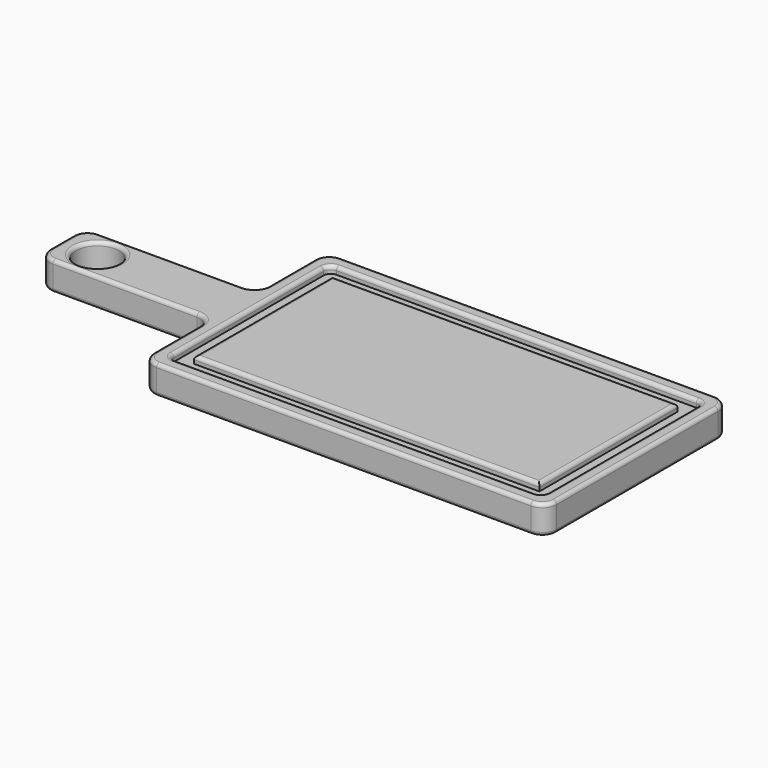
from build123d import *

# Parameters (mm, degrees)
F0_W     = 152.4
F0_H     = 50.8
F1_DEPTH = 25.4
F2_R     = 19.05
F3_DEPTH = 25.4
F5_DEPTH = 6.35
F6_R     = 6.35
F7_R     = 12.7
F8_R     = 12.7
F9_R     = 3.17499


# Not quite as in the source:
# - a fillet or chamfer is up to 0.001 mm smaller than in the source, because OpenCascade refuses the exact size


with BuildPart() as f1:
    # F0 (on Top) → F1 (new body)
    with BuildSketch(Plane.XY):
        Polygon((0, 76.2), (0, 0), (355.6, 0), (355.6, 203.2), (0, 203.2), (0, 127), align=None)
        with Locations((-76.2, 101.6)):
            Rectangle(F0_W, F0_H)
    extrude(amount=F1_DEPTH)

    # F2 (on face) → F3 (cut)
    with BuildSketch(Plane.XY.offset(25.4)):
        with Locations((-120.65, 101.6)):
            Circle(F2_R)
    extrude(amount=-F3_DEPTH, mode=Mode.SUBTRACT)

    # F4 (on face) → F5 (cut)
    with BuildSketch(Plane.XY.offset(25.4)):
        Polygon((12.6999939203, 76.2), (12.6999939203, 12.6999939203), (342.9000060797, 12.6999939203), (342.9000060797, 190.5000060797), (12.6999939203, 190.5000060797), (12.6999939203, 127), align=None)
        Polygon((25.4000002861, 76.2), (25.4000002861, 127), (25.4000002861, 177.7999997139), (330.1999997139, 177.7999997139), (330.1999997139, 25.4000002861), (25.4000002861, 25.4000002861), align=None, mode=Mode.SUBTRACT)
    extrude(amount=-F5_DEPTH, mode=Mode.SUBTRACT)

    # F6
    f6_edges = [f1.edges().sort_by_distance(p)[0] for p in [
        (12.699994, 190.500006, 22.225),
        (342.900006, 190.500006, 22.225),
        (342.900006, 12.699994, 22.225),
        (12.699994, 12.699994, 22.225),
    ]]
    fillet(f6_edges, radius=F6_R)

    # F7
    f7_edges = [f1.edges().sort_by_distance(p)[0] for p in [
        (0, 0, 12.7),
        (-152.4, 76.2, 12.7),
        (-152.4, 127, 12.7),
        (0, 203.2, 12.7),
        (355.6, 203.2, 12.7),
        (355.6, 0, 12.7),
    ]]
    fillet(f7_edges, radius=F7_R)

    # F8
    f8_edges = [f1.edges().sort_by_distance(p)[0] for p in [
        (0, 76.2, 12.7),
        (0, 127, 12.7),
    ]]
    fillet(f8_edges, radius=F8_R)

    # F9 (radius 3.175 in the source; OpenCascade refuses exactly that, so slightly less here)
    f9_edges = [f1.edges().sort_by_distance(p)[0] for p in [
        (177.8, 177.8, 25.4),
        (330.2, 101.6, 25.4),
        (177.8, 25.4, 25.4),
        (25.4, 101.6, 25.4),
        (0, 38.1, 25.4),
        (-3.719744, 72.480256, 25.4),
        (3.719744, 3.719744, 25.4),
        (-76.2, 76.2, 25.4),
        (177.8, 0, 25.4),
        (-148.680256, 79.919744, 25.4),
        (351.880256, 3.719744, 25.4),
        (-152.4, 101.6, 25.4),
        (355.6, 101.6, 25.4),
        (-148.680256, 123.280256, 25.4),
        (351.880256, 199.480256, 25.4),
        (-76.2, 127, 25.4),
        (177.8, 203.2, 25.4),
        (-3.719744, 130.719744, 25.4),
        (3.719744, 199.480256, 25.4),
        (0, 165.1, 25.4),
        (177.8, 12.699994, 25.4),
        (14.559866, 14.559866, 25.4),
        (341.040134, 14.559866, 25.4),
        (12.699994, 101.6, 25.4),
        (342.900006, 101.6, 25.4),
        (14.559866, 188.640134, 25.4),
        (341.040134, 188.640134, 25.4),
        (177.8, 190.500006, 25.4),
        (-139.7, 101.6, 25.4),
        (0, 38.1, 0),
        (-3.719744, 72.480256, 0),
        (3.719744, 3.719744, 0),
        (-76.2, 76.2, 0),
        (177.8, 0, 0),
        (-148.680256, 79.919744, 0),
        (351.880256, 3.719744, 0),
        (-152.4, 101.6, 0),
        (355.6, 101.6, 0),
        (-148.680256, 123.280256, 0),
        (351.880256, 199.480256, 0),
        (-76.2, 127, 0),
        (177.8, 203.2, 0),
        (-3.719744, 130.719744, 0),
        (3.719744, 199.480256, 0),
        (0, 165.1, 0),
        (-139.7, 101.6, 0),
    ]]
    fillet(f9_edges, radius=F9_R)


solid = f1.part
